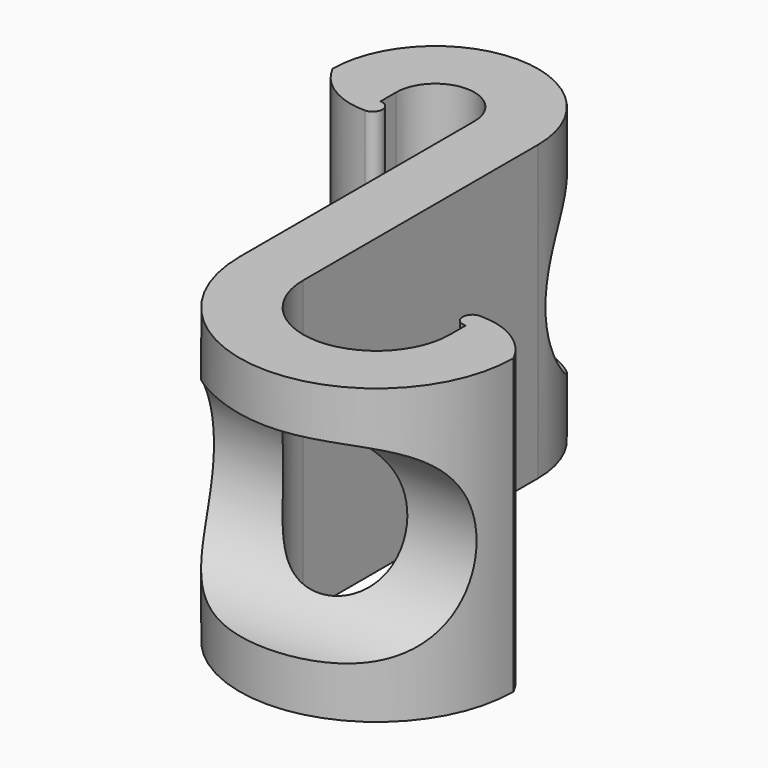
from build123d import *

# Parameters (mm, degrees)
F1_DEPTH      = 30
F3_DEPTH      = 21.001
F3_DEPTH_BACK = 21.501
F4_TEXT_SIZE  = 5.9255379407
F5_DEPTH      = 0.5


# Not quite as in the source:
# - Text() gives the source's letters only with a copy of the font that has no kerning and outlines rounded to 1/6400 em; it was checked with that copy


with BuildPart() as f1:
    # F0 (on Top) → F1 (new body)
    with BuildSketch(Plane.XY):
        with BuildLine():
            ThreePointArc((-4, 0), (0, 4), (4, 0))
            Line((4, 0), (4, -30))
            ThreePointArc((4, -30), (18, -44), (32, -30))
            ThreePointArc((32, -30), (29.3160843806, -27.0801128815), (25.5, -26))
            ThreePointArc((25.5, -26), (24.3756362681, -26.9922366967), (25.5, -27.9844733933))
            Line((25.5, -27.9844733933), (25.5, -30))
            ThreePointArc((25.5, -30), (18, -37.5), (10.5, -30))
            Line((10.5, -30), (10.5, 0))
            ThreePointArc((10.5, 0), (0, 10.5), (-10.5, 0))
            ThreePointArc((-10.5, 0), (-7.8160843806, -2.9198871185), (-4, -4))
            ThreePointArc((-4, -4), (-3, -3), (-4, -2))
            Line((-4, -2), (-4, 0))
        make_face()
    extrude(amount=F1_DEPTH)

    # F2 (on face) → F3 (cut, two sides)
    with BuildSketch(Plane.YZ.offset(10.5)) as f3_sk:
        with BuildLine():
            Line((11, 5), (11, 25))
            ThreePointArc((11, 25), (1, 15), (11, 5))
        make_face()
        with BuildLine():
            ThreePointArc((-44, 5), (-34, 15), (-44, 25))
            Line((-44, 25), (-44, 5))
        make_face()
    extrude(amount=-F3_DEPTH, mode=Mode.SUBTRACT)
    extrude(f3_sk.sketch, amount=F3_DEPTH_BACK, mode=Mode.SUBTRACT)

    # F4 (on face) → F5 (cut)
    with BuildSketch(Plane(origin=(4, 0, 0), x_dir=(0, -1, 0), z_dir=(-1, 0, 0))):
        with Locations((13.1913684309, 5.072731059)):
            Text('3E8', F4_TEXT_SIZE, font='Open Sans', text_align=(TextAlign.LEFT, TextAlign.BOTTOM))
    extrude(amount=-F5_DEPTH, mode=Mode.SUBTRACT)


solid = f1.part
